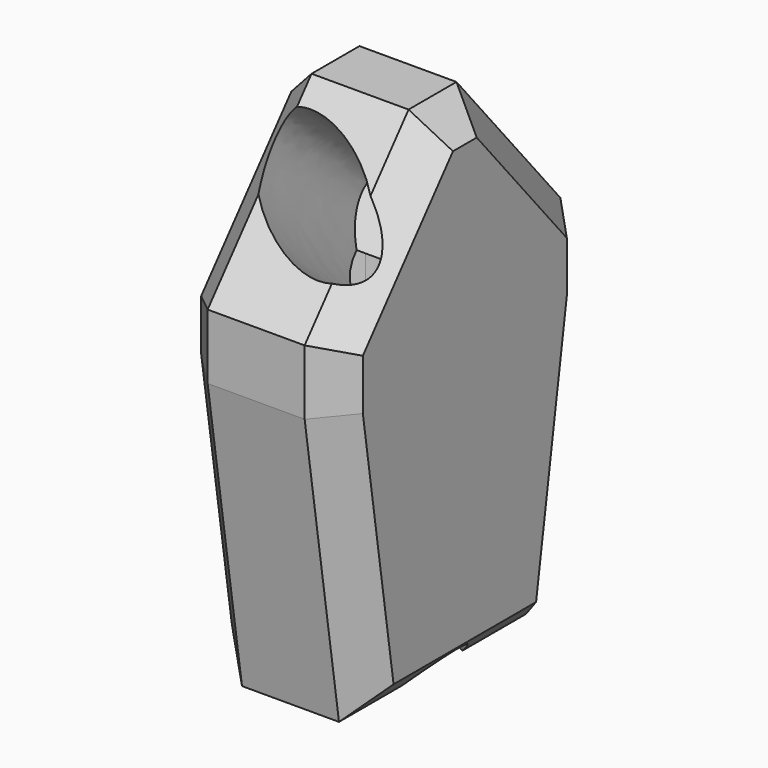
from build123d import *

# Parameters (mm, degrees)
F1_DEPTH     = 12.7
F3_DEPTH     = 25.4
F4_T1_DEPTH  = 57.8782991577
F4_T3_DEPTH  = 62.476485972
F4_T5_DEPTH  = 97.3641990785
F4_T7_DEPTH  = 35.5309018222
F4_T9_DEPTH  = 57.8782991577
F4_T11_DEPTH = 97.3641990785
F4_T13_DEPTH = 62.8567289608
F6_DEPTH     = 50.8


# Not quite as in the source:
# - a fillet or chamfer that OpenCascade refuses, or shapes differently, is made with other operations: its cross-section is extruded or revolved along the edge and cut away or added


with BuildPart() as f1:
    # F0 (on Right) → F1 (new body, symmetric)
    with BuildSketch(Plane.YZ):
        Polygon((-4.7013013323, 66.6768401792), (-25.1098079398, 42.3549291102), (-25.1098079398, 32.1350414537), (-18.3642149015, -12.4653242528), (0, -12.4653242528), (18.3642149015, -12.4653242528), (25.1098079398, 32.1350414537), (25.1098079398, 42.3549291102), (4.7013013323, 66.6768401792), (0, 66.6768401792), align=None)
    extrude(amount=F1_DEPTH, both=True)

    # F2 (on face) → F3 (cut)
    with BuildSketch(Plane(origin=(0, -35.5907714481, 29.8642031954), x_dir=(1, 0, 0), z_dir=(0, -0.7660444431, 0.6427876097))):
        with BuildLine():
            add(Edge.make_bspline(
                [(9.7735087186, 26.016607844), (17.6021152344, 35.4512603932), (-0.9724511014, 42.8986037189), (-19.5470174373, 50.3459470446), (-8.8010576172, 33.4639511697), (1.9449022029, 16.5819552948), (9.7735087186, 26.016607844)],
                knots=[0, 0, 0, 2.0943951024, 2.0943951024, 4.1887902048, 4.1887902048, 6.2831853072, 6.2831853072, 6.2831853072], degree=2, weights=[1, 0.5, 1, 0.5, 1, 0.5, 1]))
        make_face()
    extrude(amount=-F3_DEPTH, mode=Mode.SUBTRACT)

    # F4: chamfer of 5.08 on 16 edges, made by hand

    # F4_s2 → F4_t1 (cut)
    with BuildSketch(Plane(origin=(0, 39.2869435962, 46.8203561728), x_dir=(1, 0, 0), z_dir=(0, -0.6427876097, -0.7660444431))):
        Polygon((7.62, 46.4604524813), (12.7, 41.3804524813), (12.7, 46.4604524813), align=None)
        Polygon((-7.62, 46.4604524813), (-12.7, 41.3804524813), (-12.7, 46.4604524813), align=None)
    extrude(amount=F4_T1_DEPTH, mode=Mode.SUBTRACT)

    # F4_s4 → F4_t3 (cut)
    with BuildSketch(Plane.XY.offset(-7.0574072829)):
        Polygon((7.62, -25.1098079398), (12.7, -20.0298079398), (12.7, -25.1098079398), align=None)
        Polygon((12.7, 20.0298079398), (7.62, 25.1098079398), (12.7, 25.1098079398), align=None)
        Polygon((-12.7, 20.0298079398), (-7.62, 25.1098079398), (-12.7, 25.1098079398), align=None)
        Polygon((-12.7, -20.0298079398), (-7.62, -25.1098079398), (-12.7, -25.1098079398), align=None)
    extrude(amount=F4_T3_DEPTH, mode=Mode.SUBTRACT)

    # F4_s6 → F4_t5 (cut)
    with BuildSketch(Plane(origin=(0, -11.1741383172, 73.8809253053), x_dir=(1, 0, 0), z_dir=(0, 0.1495444875, -0.9887549981))):
        Polygon((12.7, 14.9418297969), (7.62, 20.0218297969), (12.7, 20.0218297969), align=None)
        Polygon((-12.7, 14.9418297969), (-7.62, 20.0218297969), (-12.7, 20.0218297969), align=None)
    extrude(amount=F4_T5_DEPTH, mode=Mode.SUBTRACT)

    # F4_s8 → F4_t7 (cut)
    with BuildSketch(Plane.XZ.offset(-17.7654509111)):
        Polygon((7.62, 66.6768401792), (12.7, 61.5968401792), (12.7, 66.6768401792), align=None)
        Polygon((-12.7, 61.5968401792), (-7.62, 66.6768401792), (-12.7, 66.6768401792), align=None)
    extrude(amount=F4_T7_DEPTH, mode=Mode.SUBTRACT)

    # F4_s10 → F4_t9 (cut)
    with BuildSketch(Plane(origin=(0, -2.0834900279, 2.4830067258), x_dir=(1, 0, 0), z_dir=(0, -0.6427876097, 0.7660444431))):
        Polygon((12.7, 41.3804524813), (7.62, 46.4604524813), (12.7, 46.4604524813), align=None)
        Polygon((-12.7, 41.3804524813), (-7.62, 46.4604524813), (-12.7, 46.4604524813), align=None)
    extrude(amount=F4_T9_DEPTH, mode=Mode.SUBTRACT)

    # F4_s12 → F4_t11 (cut)
    with BuildSketch(Plane(origin=(0, -3.3861409345, -22.3884131691), x_dir=(1, 0, 0), z_dir=(0, 0.1495444875, 0.9887549981))):
        Polygon((12.7, 14.9418297969), (7.62, 20.0218297969), (12.7, 20.0218297969), align=None)
        Polygon((-12.7, 14.9418297969), (-7.62, 20.0218297969), (-12.7, 20.0218297969), align=None)
    extrude(amount=F4_T11_DEPTH, mode=Mode.SUBTRACT)

    # F4_s14 → F4_t13 (cut)
    with BuildSketch(Plane.XZ.offset(-31.4283644804)):
        Polygon((12.7, -7.3853242528), (7.62, -12.4653242528), (12.7, -12.4653242528), align=None)
        Polygon((-12.7, -7.3853242528), (-7.62, -12.4653242528), (-12.7, -12.4653242528), align=None)
    extrude(amount=F4_T13_DEPTH, mode=Mode.SUBTRACT)

    # F5 (on face) → F6 (cut)
    with BuildSketch(Plane(origin=(0, 0, -12.4653242528), x_dir=(1, 0, 0), z_dir=(0, 0, -1))):
        with BuildLine():
            Line((-7.62, 5.8784427825), (-7.62, -5.8784427825))
            add(Edge.make_bspline(
                [(-7.62, -5.8784427825), (0, -10.3327032159), (7.62, -5.8784427825)],
                knots=[0.8545345114, 0.8545345114, 0.8545345114, 2.2870581422, 2.2870581422, 2.2870581422], degree=2, weights=[1, 0.7542653721, 1]))
            Line((7.62, -5.8784427825), (7.62, 5.8784427825))
            add(Edge.make_bspline(
                [(7.62, 5.8784427825), (0, 10.3327032159), (-7.62, 5.8784427825)],
                knots=[3.9961271649, 3.9961271649, 3.9961271649, 5.4286507958, 5.4286507958, 5.4286507958], degree=2, weights=[1, 0.7542653721, 1]))
        make_face()
        with BuildLine():
            add(Edge.make_bspline(
                [(-7.62, 5.8784427825), (-11.6057749838, 3.5485635427), (-11.6057749838, 0)],
                knots=[5.4286507958, 5.4286507958, 5.4286507958, 6.2831853072, 6.2831853072, 6.2831853072], degree=2, weights=[1, 0.9101015555, 1]))
            add(Edge.make_bspline(
                [(-11.6057749838, 0), (-11.6057749838, -3.5485635427), (-7.62, -5.8784427825)],
                knots=[0, 0, 0, 0.8545345114, 0.8545345114, 0.8545345114], degree=2, weights=[1, 0.9101015555, 1]))
            Line((-7.62, -5.8784427825), (-7.62, 5.8784427825))
        make_face()
        with BuildLine():
            Line((7.62, 5.8784427825), (7.62, -5.8784427825))
            add(Edge.make_bspline(
                [(7.62, -5.8784427825), (17.6763796553, 0), (7.62, 5.8784427825)],
                knots=[2.2870581422, 2.2870581422, 2.2870581422, 3.9961271649, 3.9961271649, 3.9961271649], degree=2, weights=[1, 0.6565696828, 1]))
        make_face()
    extrude(amount=-F6_DEPTH, mode=Mode.SUBTRACT)


solid = f1.part
